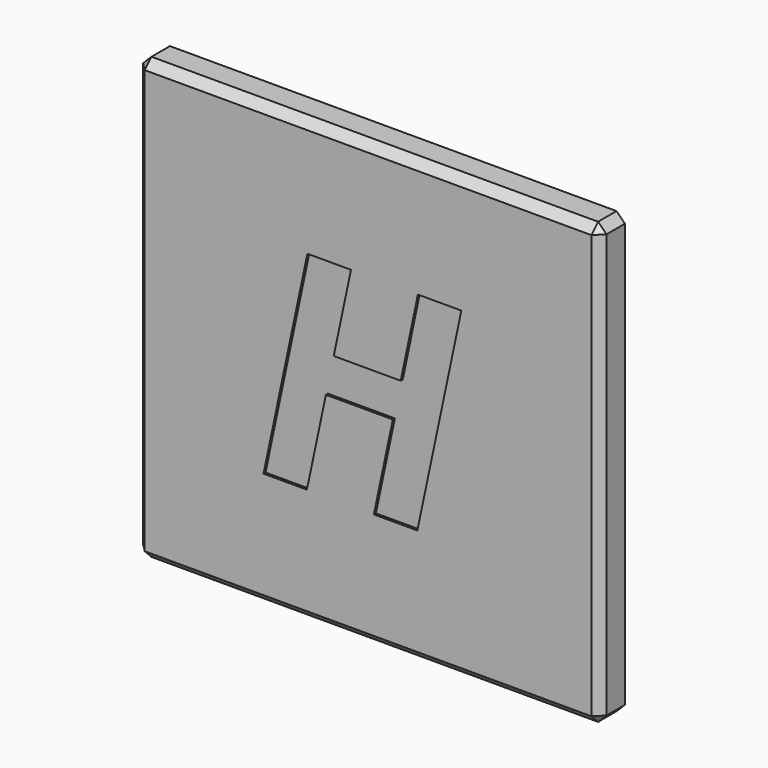
from build123d import *

# Parameters (mm, degrees)
F1_W         = 110.5
F1_H         = 105
F2_DEPTH     = 7.5
F0_W         = 106.5
F0_H         = 101
F3_DEPTH     = 2.6
F4_W         = 96.5
F4_H         = 91
F5_DEPTH     = 5.5
F6_TEXT_SIZE = 69.4444444444
F7_DEPTH     = 0.6
F8_SIZE      = 2


# Not quite as in the source:
# - Text() gives the source's letters only with a copy of the font that has no kerning and outlines rounded to 1/6400 em; it was checked with that copy


with BuildPart() as f2:
    # F1 (on Front) → F2 (new body)
    with BuildSketch(Plane.XZ):
        Rectangle(F1_W, F1_H)
    extrude(amount=F2_DEPTH)

    # F0 (on Front) → F3 (cut)
    with BuildSketch(Plane.XZ):
        Rectangle(F0_W, F0_H)
    extrude(amount=F3_DEPTH, mode=Mode.SUBTRACT)

    # F4 (on Front) → F5 (cut)
    with BuildSketch(Plane.XZ):
        Rectangle(F4_W, F4_H)
    extrude(amount=F5_DEPTH, mode=Mode.SUBTRACT)

    # F6 (on face) → F7 (cut)
    with BuildSketch(Plane.XZ.offset(7.5)):
        with Locations((-26.7361111111, -25)):
            Text('H', F6_TEXT_SIZE, font='Open Sans', font_style=FontStyle.BOLDITALIC, text_align=(TextAlign.LEFT, TextAlign.BOTTOM))
    extrude(amount=-F7_DEPTH, mode=Mode.SUBTRACT)

    # F8
    f8_edges = [f2.edges().sort_by_distance(p)[0] for p in [
        (55.25, -3.75, 52.5),
        (-55.25, -3.75, 52.5),
        (55.25, -3.75, -52.5),
        (-55.25, -3.75, -52.5),
        (0, -7.5, -52.5),
        (-55.25, -7.5, 0),
        (0, -7.5, 52.5),
        (55.25, -7.5, 0),
    ]]
    chamfer(f8_edges, length=F8_SIZE)


solid = f2.part
